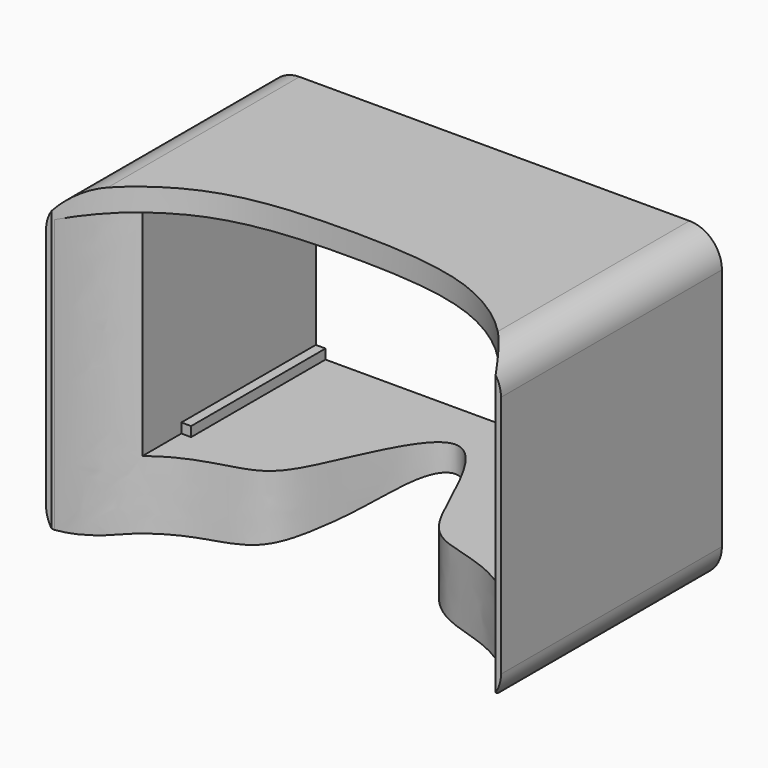
from build123d import *

# Parameters (mm, degrees)
F0_W      = 140
F0_H      = 170
F1_DEPTH  = 95
F2_W      = 110
F2_H      = 67
F3_DEPTH  = 170.001
F5_DEPTH  = 88
F7_DEPTH  = 95.001
F8_R      = 10
F10_DEPTH = 170.001
F11_W     = 121
F11_H     = 76
F11_W_2   = 110
F11_H_2   = 67
F12_DEPTH = 3
F13_W     = 3
F13_H     = 90
F14_DEPTH = 3
F15_W     = 3
F15_H     = 90
F16_DEPTH = 3
F17_R     = 1.3
F18_DEPTH = 100
F19_R     = 3.1
F20_DEPTH = 75
F21_W     = 145
F21_H     = 85
F22_DEPTH = 95.001


with BuildPart() as f1:
    # F0 (on Top) → F1 (new body)
    with BuildSketch(Plane.XY):
        Rectangle(F0_W, F0_H)
    extrude(amount=F1_DEPTH)

    # F2 (on face) → F3 (cut, through all)
    with BuildSketch(Plane.XZ.offset(85)):
        with Locations((0, 54.5)):
            Rectangle(F2_W, F2_H)
    extrude(amount=-F3_DEPTH, mode=Mode.SUBTRACT)

    # F4 (on face) → F5 (cut)
    with BuildSketch(Plane(origin=(0, 0, 0), x_dir=(1, 0, 0), z_dir=(0, 0, -1))):
        with BuildLine():
            add(Edge.make_bspline(
                [(0, 15), (-7.79441, 15), (-19.466411, 48.056936), (-30.975012, 59.107625), (-57.856268, 61.12551), (-68.258241, 85)],
                knots=[0, 0, 0, 0, 0.355883, 0.597297, 1, 1, 1, 1], degree=3))
            add(Edge.make_bspline(
                [(0, 15), (7.79441, 15), (19.466411, 48.056936), (30.975012, 59.107625), (57.856268, 61.12551), (68.258241, 85)],
                knots=[0, 0, 0, 0, 0.355883, 0.597297, 1, 1, 1, 1], degree=3))
            Line((68.258241, 85), (-68.258241, 85))
        make_face()
    extrude(amount=-F5_DEPTH, mode=Mode.SUBTRACT)

    # F6 (on face) → F7 (cut, through all)
    with BuildSketch(Plane.XY.offset(95)):
        with BuildLine():
            add(Edge.make_bspline(
                [(0, -55), (25.389496, -55), (47.041007, -60.614282), (62.843867, -75.413413), (68.355819, -85)],
                knots=[0, 0, 0, 0, 0.564508, 1, 1, 1, 1], degree=3))
            add(Edge.make_bspline(
                [(0, -55), (-25.389496, -55), (-47.041007, -60.614282), (-62.843867, -75.413413), (-68.355819, -85)],
                knots=[0, 0, 0, 0, 0.564508, 1, 1, 1, 1], degree=3))
            Line((-68.355819, -85), (68.355819, -85))
        make_face()
    extrude(amount=-F7_DEPTH, mode=Mode.SUBTRACT)

    # F8
    f8_edges = [f1.edges().sort_by_distance(p)[0] for p in [
        (70, 0, 95),
        (70, 0, 0),
        (-70, 0, 0),
        (-70, 0, 95),
    ]]
    fillet(f8_edges, radius=F8_R)

    # F9 (on face) → F10 (cut, through all)
    with BuildSketch(Plane(origin=(0, 85, 0), x_dir=(-1, 0, 0), z_dir=(0, 1, 0))):
        with BuildLine():
            add(Edge.make_bspline(
                [(0, 13), (14.179069, 13), (11.016984, 0), (40, 0)],
                knots=[0, 0, 0, 0, 42.059482, 42.059482, 42.059482, 42.059482], degree=3))
            add(Edge.make_bspline(
                [(0, 13), (-14.179069, 13), (-11.016984, 0), (-40, 0)],
                knots=[0, 0, 0, 0, 42.059482, 42.059482, 42.059482, 42.059482], degree=3))
            Line((-40, 0), (40, 0))
        make_face()
    extrude(amount=-F10_DEPTH, mode=Mode.SUBTRACT)

    # F11 (on face) → F12 (cut)
    with BuildSketch(Plane(origin=(0, 85, 0), x_dir=(-1, 0, 0), z_dir=(0, 1, 0))):
        with Locations((0, 52)):
            Rectangle(F11_W, F11_H)
        with Locations((0, 54.5)):
            Rectangle(F11_W_2, F11_H_2, mode=Mode.SUBTRACT)
    extrude(amount=-F12_DEPTH, mode=Mode.SUBTRACT)

    # F13 (on face) → F14 (join)
    with BuildSketch(Plane.XY.offset(21)):
        with Locations((-53.5, -6.706829)):
            Rectangle(F13_W, F13_H)
        with Locations((53.5, -6.706829)):
            Rectangle(F13_W, F13_H)
    extrude(amount=F14_DEPTH)

    # F15 (on face) → F16 (join)
    with BuildSketch(Plane(origin=(0, 0, 88), x_dir=(1, 0, 0), z_dir=(0, 0, -1))):
        with Locations((53.5, 6.706829)):
            Rectangle(F15_W, F15_H)
        with Locations((-53.5, 6.706829)):
            Rectangle(F15_W, F15_H)
    extrude(amount=F16_DEPTH)

    # F17 (on face) → F18 (cut)
    with BuildSketch(Plane(origin=(0, 85, 0), x_dir=(-1, 0, 0), z_dir=(0, 1, 0))):
        with Locations((65, 77.5)):
            Circle(F17_R)
        with Locations((65, 17.5)):
            Circle(F17_R)
        with Locations((-65, 77.5)):
            Circle(F17_R)
        with Locations((-65, 17.5)):
            Circle(F17_R)
    extrude(amount=-F18_DEPTH, mode=Mode.SUBTRACT)

    # F19 (on face) → F20 (cut)
    with BuildSketch(Plane(origin=(0, 85, 0), x_dir=(-1, 0, 0), z_dir=(0, 1, 0))):
        with Locations((65, 77.5)):
            Circle(F19_R)
        with Locations((65, 17.5)):
            Circle(F19_R)
        with Locations((-65, 77.5)):
            Circle(F19_R)
        with Locations((-65, 17.5)):
            Circle(F19_R)
    extrude(amount=-F20_DEPTH, mode=Mode.SUBTRACT)

    # F21 (on face) → F22 (cut, through all)
    with BuildSketch(Plane.XY.offset(95)):
        with Locations((-0.091513, 42.5)):
            Rectangle(F21_W, F21_H)
    extrude(amount=-F22_DEPTH, mode=Mode.SUBTRACT)


solid = f1.part
